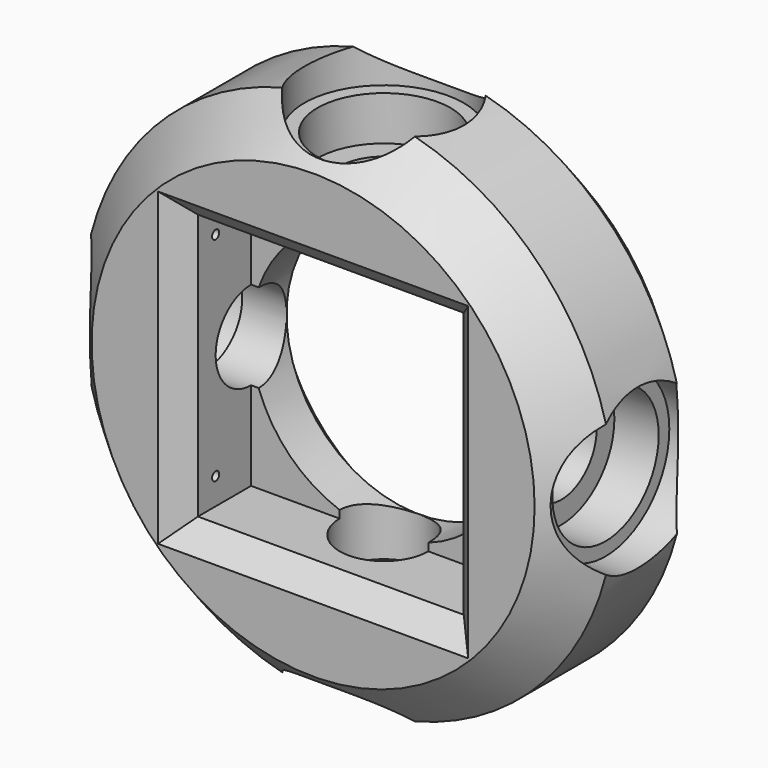
from build123d import *

# Parameters (mm, degrees)
F0_R      = 30
F0_R_2    = 15
F1_DEPTH  = 10
F4_R      = 5
F5_DEPTH  = 77.4
F6_R      = 7.5
F7_DEPTH  = 10
F8_R      = 9
F9_DEPTH  = 5
F10_R     = 7.5
F11_DEPTH = 10
F12_R     = 9
F13_DEPTH = 5
F16_R     = 7.5
F17_DEPTH = 10
F18_R     = 5
F19_DEPTH = 88.4
F20_R     = 9
F21_DEPTH = 5
F22_R     = 7.5
F23_DEPTH = 10
F24_R     = 9
F25_DEPTH = 5
F26_W     = 30
F26_H     = 30
F27_DEPTH = 21.4
F28_R     = 0.5
F29_DEPTH = 17.5
F30_R     = 0.5
F31_DEPTH = 17.5
F34_SIZE  = 4.99999
F35_SIZE  = 2.5
F36_SIZE  = 2.5
F37_SIZE  = 2.5


# Not quite as in the source:
# - a fillet or chamfer that OpenCascade refuses, or shapes differently, is made with other operations: its cross-section is extruded or revolved along the edge and cut away or added
# - a fillet or chamfer is up to 0.001 mm smaller than in the source, because OpenCascade refuses the exact size


with BuildPart() as f1:
    # F0 (on Front) → F1 (new body, symmetric)
    with BuildSketch(Plane.XZ):
        Circle(F0_R)
        Circle(F0_R_2, mode=Mode.SUBTRACT)
    extrude(amount=F1_DEPTH, both=True)

    # F4 (on offset) → F5 (cut)
    with BuildSketch(Plane.XY.offset(-30)):
        Circle(F4_R)
    extrude(amount=F5_DEPTH, mode=Mode.SUBTRACT)

    # F6 (on offset) → F7 (cut)
    with BuildSketch(Plane.XY.offset(30)):
        Circle(F6_R)
    extrude(amount=-F7_DEPTH, mode=Mode.SUBTRACT)

    # F8 (on offset) → F9 (cut)
    with BuildSketch(Plane.XY.offset(30)):
        Circle(F8_R)
    extrude(amount=-F9_DEPTH, mode=Mode.SUBTRACT)

    # F10 (on offset) → F11 (cut)
    with BuildSketch(Plane.XY.offset(-30)):
        Circle(F10_R)
    extrude(amount=F11_DEPTH, mode=Mode.SUBTRACT)

    # F12 (on offset) → F13 (cut)
    with BuildSketch(Plane.XY.offset(-30)):
        Circle(F12_R)
    extrude(amount=F13_DEPTH, mode=Mode.SUBTRACT)

    # F16 (on offset) → F17 (cut)
    with BuildSketch(Plane.YZ.offset(30)):
        Circle(F16_R)
    extrude(amount=-F17_DEPTH, mode=Mode.SUBTRACT)

    # F18 (on offset) → F19 (cut)
    with BuildSketch(Plane.YZ.offset(30)):
        Circle(F18_R)
    extrude(amount=-F19_DEPTH, mode=Mode.SUBTRACT)

    # F20 (on offset) → F21 (cut)
    with BuildSketch(Plane.YZ.offset(30)):
        Circle(F20_R)
    extrude(amount=-F21_DEPTH, mode=Mode.SUBTRACT)

    # F22 (on offset) → F23 (cut)
    with BuildSketch(Plane.YZ.offset(-30)):
        Circle(F22_R)
    extrude(amount=F23_DEPTH, mode=Mode.SUBTRACT)

    # F24 (on offset) → F25 (cut)
    with BuildSketch(Plane.YZ.offset(-30)):
        Circle(F24_R)
    extrude(amount=F25_DEPTH, mode=Mode.SUBTRACT)

    # F26 (on Front) → F27 (cut)
    with BuildSketch(Plane.XZ):
        Rectangle(F26_W, F26_H)
    extrude(amount=F27_DEPTH, mode=Mode.SUBTRACT)

    # F28 (on Right) → F29 (cut, symmetric)
    with BuildSketch(Plane.YZ):
        with Locations((-5, 12)):
            Circle(F28_R)
        with Locations((-5, -12)):
            Circle(F28_R)
    extrude(amount=F29_DEPTH, both=True, mode=Mode.SUBTRACT)

    # F30 (on Right) → F31 (cut, symmetric)
    with BuildSketch(Plane.YZ):
        with Locations((-5, -12)):
            Circle(F30_R)
    extrude(amount=F31_DEPTH, both=True, mode=Mode.SUBTRACT)

    # F32: chamfer of 5 on 1 edges, made by hand

    # F32_s1 → F32_t2 (revolve, cut)
    with BuildSketch(Plane.XY):
        Polygon((30, 5), (25, 10), (30, 10), align=None)
    revolve(axis=Axis((0, 10, 0), (0, -1, 0)), mode=Mode.SUBTRACT)

    # F33: chamfer of 5 on 1 edges, made by hand

    # F33_s1 → F33_t2 (revolve, cut)
    with BuildSketch(Plane.XY):
        Polygon((30, -5), (25, -10), (30, -10), align=None)
    revolve(axis=Axis((0, -10, 0), (0, -1, 0)), mode=Mode.SUBTRACT)

    # F34 (size 5 in the source; OpenCascade refuses exactly that, so slightly less here)
    f34_edges = [f1.edges().sort_by_distance(p)[0] for p in [
        (-15, 10, 0),
    ]]
    chamfer(f34_edges, length=F34_SIZE)

    # F35
    f35_edges = [f1.edges().sort_by_distance(p)[0] for p in [
        (0, -10, -15),
    ]]
    chamfer(f35_edges, length=F35_SIZE)

    # F36
    f36_edges = [f1.edges().sort_by_distance(p)[0] for p in [
        (15, -10, 0),
    ]]
    chamfer(f36_edges, length=F36_SIZE)

    # F37
    f37_edges = [f1.edges().sort_by_distance(p)[0] for p in [
        (0, -10, 15),
        (-15, -10, 0),
    ]]
    chamfer(f37_edges, length=F37_SIZE)


solid = f1.part
